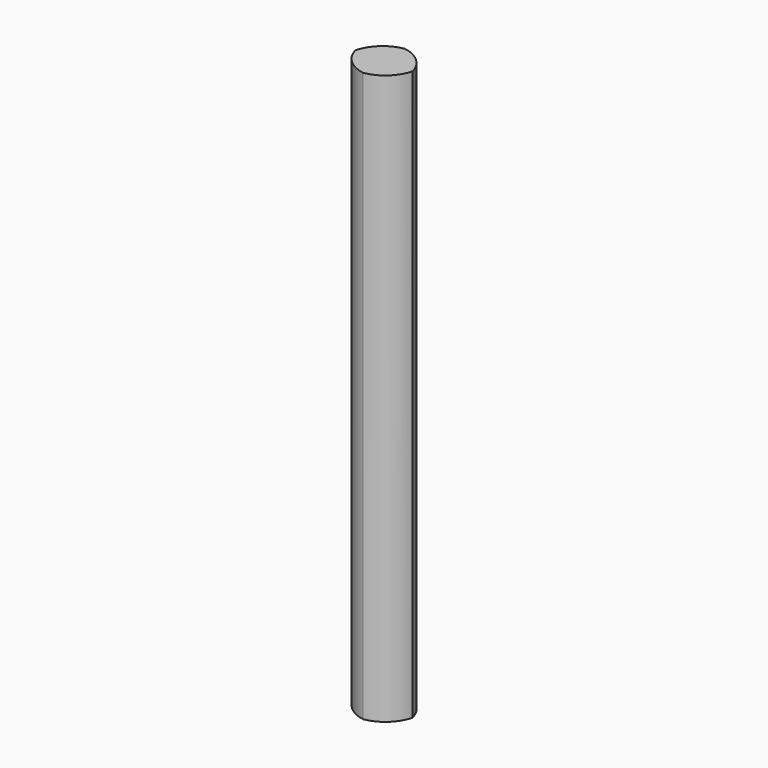
from build123d import *

# Parameters (mm, degrees)
F0_W        = 8.5262348875
F0_H        = 81.7743241787
F1_DEPTH    = 3.81
F2_T1_DEPTH = 107.1743241787


# Not quite as in the source:
# - a fillet or chamfer that OpenCascade refuses, or shapes differently, is made with other operations: its cross-section is extruded or revolved along the edge and cut away or added


with BuildPart() as f1:
    # F0 (on Front) → F1 (new body, symmetric)
    with BuildSketch(Plane.XZ):
        with Locations((0.1593702473, -1.1174529791)):
            Rectangle(F0_W, F0_H)
    extrude(amount=F1_DEPTH, both=True)

    # F2: fillet of radius 5.08 on 4 edges, made by hand

    # F2_s2 → F2_t1 (cut)
    with BuildSketch(Plane.XY.offset(-54.7046150684)):
        with BuildLine():
            ThreePointArc((4.422487691, 1.27), (2.9345901395, -2.3221024484), (-0.657512309, -3.81))
            Line((-0.657512309, -3.81), (4.422487691, -3.81))
            Line((4.422487691, -3.81), (4.422487691, 1.27))
        make_face()
        with BuildLine():
            ThreePointArc((4.422487691, -1.27), (2.9345901395, 2.3221024484), (-0.657512309, 3.81))
            Line((-0.657512309, 3.81), (4.422487691, 3.81))
            Line((4.422487691, 3.81), (4.422487691, -1.27))
        make_face()
        with BuildLine():
            ThreePointArc((-4.1037471965, 1.27), (-2.6158496449, -2.3221024484), (0.9762528035, -3.81))
            Line((0.9762528035, -3.81), (-4.1037471965, -3.81))
            Line((-4.1037471965, -3.81), (-4.1037471965, 1.27))
        make_face()
        with BuildLine():
            ThreePointArc((-4.1037471965, -1.27), (-2.6158496449, 2.3221024484), (0.9762528035, 3.81))
            Line((0.9762528035, 3.81), (-4.1037471965, 3.81))
            Line((-4.1037471965, 3.81), (-4.1037471965, -1.27))
        make_face()
    extrude(amount=F2_T1_DEPTH, mode=Mode.SUBTRACT)


solid = f1.part
